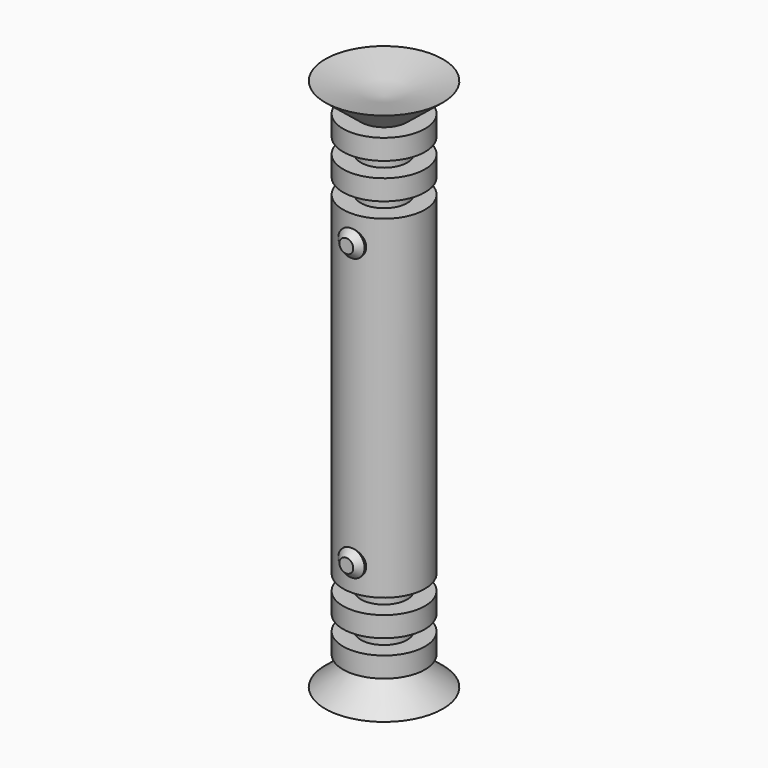
from build123d import *

# Parameters (mm, degrees)
F2_R         = 10.6813712462
F3_DEPTH     = 38.1
F4_S5_R      = 33.1123778597
F4_T6_DEPTH  = 17
F4_S11_R     = 33.1123778597
F4_T12_DEPTH = 17


# Not quite as in the source:
# - a fillet or chamfer that OpenCascade refuses, or shapes differently, is made with other operations: its cross-section is extruded or revolved along the edge and cut away or added


with BuildPart() as f1:
    # F0 (on Front) → F1 (revolve)
    with BuildSketch(Plane.XZ):
        Polygon((33.1123778597, 0), (0, 0), (0, -204.5256793499), (47.4873222411, -215.4780179262), (18.7374334782, -192.2043114901), (33.1123778597, -192.2043114901), (33.1123778597, -175.7757812738), (18.7374334782, -175.7757812738), (18.7374334782, -163.4543985128), (33.1123778597, -163.4543985128), (33.1123778597, -147.0258831978), (18.7374334782, -147.0258831978), (18.7374334782, -134.7045004368), (33.1123778597, -134.7045004368), align=None)
        Polygon((0, 204.5256793499), (0, 0), (33.1123778597, 0), (33.1123778597, 134.7045004368), (18.7374334782, 134.7045004368), (18.7374334782, 147.0258831978), (33.1123778597, 147.0258831978), (33.1123778597, 163.4543985128), (18.7374334782, 163.4543985128), (18.7374334782, 175.7757812738), (33.1123778597, 175.7757812738), (33.1123778597, 192.2043114901), (18.7374334782, 192.2043114901), (47.4873222411, 215.4780179262), align=None)
    revolve(axis=Axis((0, 0, -102.2628396749), (0, 0, -1)))

    # F2 (on Front) → F3 (join)
    with BuildSketch(Plane.XZ):
        with Locations((0, 113.5328859091)):
            Circle(F2_R)
        with Locations((0, -113.5328859091)):
            Circle(F2_R)
    extrude(amount=F3_DEPTH)

    # F4: chamfer of 5.08 on 2 edges, made by hand


with BuildPart() as f4_tool2:
    # F4_s3 → F4_t4 (revolve)
    with BuildSketch(Plane.XY.offset(113.5328859091)):
        Polygon((10.6813712462, -33.02), (5.6013712462, -38.1), (10.6813712462, -38.1), align=None)
    revolve(axis=Axis((0, -38.1, 113.5328859091), (0, -1, 0)))

    # F4_s5 → F4_t6 (cut, symmetric)
    with BuildSketch(Plane.XY.offset(113.5)):
        Circle(F4_S5_R)
    extrude(amount=F4_T6_DEPTH, both=True, mode=Mode.SUBTRACT)


with BuildPart() as f1_1:
    add(f1.part)

    # F4_t1: cut F4_tool2
    add(f4_tool2.part, mode=Mode.SUBTRACT)


with BuildPart() as f4_tool8:
    # F4_s9 → F4_t10 (revolve)
    with BuildSketch(Plane.XY.offset(-113.5328859091)):
        Polygon((10.6813712462, -33.02), (5.6013712462, -38.1), (10.6813712462, -38.1), align=None)
    revolve(axis=Axis((0, -38.1, -113.5328859091), (0, -1, 0)))

    # F4_s11 → F4_t12 (cut, symmetric)
    with BuildSketch(Plane.XY.offset(-113.5)):
        Circle(F4_S11_R)
    extrude(amount=F4_T12_DEPTH, both=True, mode=Mode.SUBTRACT)


with BuildPart() as f1_2:
    add(f1_1.part)

    # F4_t7: cut F4_tool8
    add(f4_tool8.part, mode=Mode.SUBTRACT)


solid = f1_2.part
